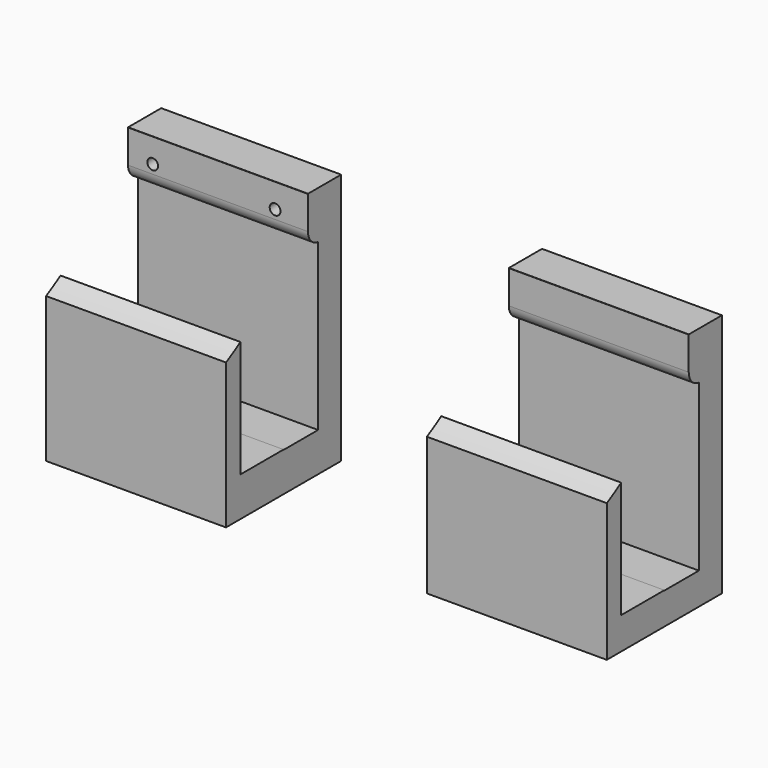
from build123d import *

# Parameters (mm, degrees)
F0_W           = 63.5
F0_H           = 203.2
F1_DEPTH       = 25.4
F2_R           = 5.08
F2_2_R         = 5.08
F3_R           = 85.5041731658
F4_DEPTH       = 152.4
F5_W           = 19.05
F5_H           = 58.3084138111
F6_DEPTH       = 190.5
F7_W           = 15.24
F7_H           = 58.42
F8_DEPTH       = 190.5
F9_R           = 5.08
F9_2_R         = 5.08
F10_W          = 137.1934004128
F10_H          = 115.8126294613
F11_DEPTH      = 635
F12_W          = 13.0418678746
F12_H          = 28.3660627902
F13_DEPTH      = 254
F14_W          = 37.495367229
F14_H          = 80.2074819803
F15_DEPTH      = 254
F16_R          = 1.905
F17_DEPTH      = 127
F18_T1_DEPTH   = 88.7224853994
F18_2_T1_DEPTH = 88.7224853994


# Not quite as in the source:
# - a fillet or chamfer that OpenCascade refuses, or shapes differently, is made with other operations: its cross-section is extruded or revolved along the edge and cut away or added


with BuildPart() as f1:
    # F0 (on Front) → F1 (new body, symmetric)
    with BuildSketch(Plane.XZ):
        with Locations((-102.6535956171, 29.415011573)):
            Rectangle(F0_W, F0_H)
    extrude(amount=F1_DEPTH, both=True)

    # F2
    f2_edges = [f1.edges().sort_by_distance(p)[0] for p in [
        (-102.653596, -25.4, 131.015012),
    ]]
    fillet(f2_edges, radius=F2_R)


with BuildPart() as f1b:
    # F0 (on Front) → F1, piece 2 (new body, symmetric)
    with BuildSketch(Plane.XZ):
        with Locations((31.75, 31.9777971928)):
            Rectangle(F0_W, F0_H)
    extrude(amount=F1_DEPTH, both=True)

    # F2#2
    f2_2_edges = [f1b.edges().sort_by_distance(p)[0] for p in [
        (31.75, -25.4, 133.577797),
    ]]
    fillet(f2_2_edges, radius=F2_2_R)


with BuildPart() as f4_tool:
    # F3 (on Right) → F4 (new body, symmetric)
    with BuildSketch(Plane.YZ):
        with Locations((-66.0597089804, 54.2870010056)):
            Circle(F3_R)
    extrude(amount=F4_DEPTH, both=True)


with BuildPart() as f1_1:
    add(f1.part)

    # F4: cut by f4_tool
    add(f4_tool.part, mode=Mode.SUBTRACT)


with BuildPart() as f1b_1:
    add(f1b.part)

    # F4: cut by f4_tool
    add(f4_tool.part, mode=Mode.SUBTRACT)


with BuildPart() as f6_tool:
    # F5 (on Right) → F6 (new body, symmetric)
    with BuildSketch(Plane.YZ):
        with Locations((-9.525, -29.1542069055)):
            Rectangle(F5_W, F5_H)
    extrude(amount=F6_DEPTH, both=True)


with BuildPart() as f1_2:
    add(f1_1.part)

    # F6: cut by f6_tool
    add(f6_tool.part, mode=Mode.SUBTRACT)


with BuildPart() as f1b_2:
    add(f1b_1.part)

    # F6: cut by f6_tool
    add(f6_tool.part, mode=Mode.SUBTRACT)


with BuildPart() as f8_tool:
    # F7 (on Right) → F8 (new body, symmetric)
    with BuildSketch(Plane.YZ):
        with Locations((7.62, -29.21)):
            Rectangle(F7_W, F7_H)
    extrude(amount=F8_DEPTH, both=True)


with BuildPart() as f1_3:
    add(f1_2.part)

    # F8: cut by f8_tool
    add(f8_tool.part, mode=Mode.SUBTRACT)

    # F9
    f9_edges = [f1_3.edges().sort_by_distance(p)[0] for p in [
        (-102.653596, 0, 0),
    ]]
    fillet(f9_edges, radius=F9_R)


with BuildPart() as f1b_3:
    add(f1b_2.part)

    # F8: cut by f8_tool
    add(f8_tool.part, mode=Mode.SUBTRACT)

    # F9#2
    f9_2_edges = [f1b_3.edges().sort_by_distance(p)[0] for p in [
        (31.75, 0, 0),
    ]]
    fillet(f9_2_edges, radius=F9_2_R)


with BuildPart() as f11_tool:
    # F10 (on Right) → F11 (new body, symmetric)
    with BuildSketch(Plane.YZ):
        with Locations((25.8351210505, 135.2587789297)):
            Rectangle(F10_W, F10_H)
    extrude(amount=F11_DEPTH, both=True)


with BuildPart() as f1_4:
    add(f1_3.part)

    # F11: cut by f11_tool
    add(f11_tool.part, mode=Mode.SUBTRACT)


with BuildPart() as f1b_4:
    add(f1b_3.part)

    # F11: cut by f11_tool
    add(f11_tool.part, mode=Mode.SUBTRACT)


with BuildPart() as f13_tool:
    # F12 (on Right) → F13 (new body, symmetric)
    with BuildSketch(Plane.YZ):
        with Locations((4.2386068963, 4.7333268449)):
            Rectangle(F12_W, F12_H)
    extrude(amount=F13_DEPTH, both=True)


with BuildPart() as f1_5:
    add(f1_4.part)

    # F13: cut by f13_tool
    add(f13_tool.part, mode=Mode.SUBTRACT)


with BuildPart() as f1b_5:
    add(f1b_4.part)

    # F13: cut by f13_tool
    add(f13_tool.part, mode=Mode.SUBTRACT)


with BuildPart() as f15_tool:
    # F14 (on Right) → F15 (new body, symmetric)
    with BuildSketch(Plane.YZ):
        with Locations((22.6602442563, 56.9007955492)):
            Rectangle(F14_W, F14_H)
    extrude(amount=F15_DEPTH, both=True)


with BuildPart() as f1_6:
    add(f1_5.part)

    # F15: cut by f15_tool
    add(f15_tool.part, mode=Mode.SUBTRACT)

    # F16 (on Front) → F17 (cut, symmetric)
    with BuildSketch(Plane.XZ):
        with Locations((-125.6962865591, 8.1708896905)):
            Circle(F16_R)
        with Locations((-82.4957340956, 8.1708896905)):
            Circle(F16_R)
    extrude(amount=F17_DEPTH, both=True, mode=Mode.SUBTRACT)

    # F18: fillet of radius 5.08 on 1 edges, made by hand

    # F18_s2 → F18_t1 (cut)
    with BuildSketch(Plane.YZ.offset(-147.0148383168)):
        with BuildLine():
            ThreePointArc((10.7595408335, 5.0444970799), (12.0413789469, 1.6710172322), (15.24, 0))
            Line((15.24, 0), (10.7595408335, 0))
            Line((10.7595408335, 0), (10.7595408335, 5.0444970799))
        make_face()
    extrude(amount=F18_T1_DEPTH, mode=Mode.SUBTRACT)


with BuildPart() as f1b_6:
    add(f1b_5.part)

    # F15: cut by f15_tool
    add(f15_tool.part, mode=Mode.SUBTRACT)

    # F18#2: fillet of radius 5.08 on 1 edges, made by hand

    # F18_2_s2 → F18_2_t1 (cut)
    with BuildSketch(Plane.YZ.offset(-12.6112426997)):
        with BuildLine():
            ThreePointArc((10.7595408335, 5.0444970799), (12.0413789469, 1.6710172322), (15.24, 0))
            Line((15.24, 0), (10.7595408335, 0))
            Line((10.7595408335, 0), (10.7595408335, 5.0444970799))
        make_face()
    extrude(amount=F18_2_T1_DEPTH, mode=Mode.SUBTRACT)


solid = Compound([f1_6.part, f1b_6.part])
